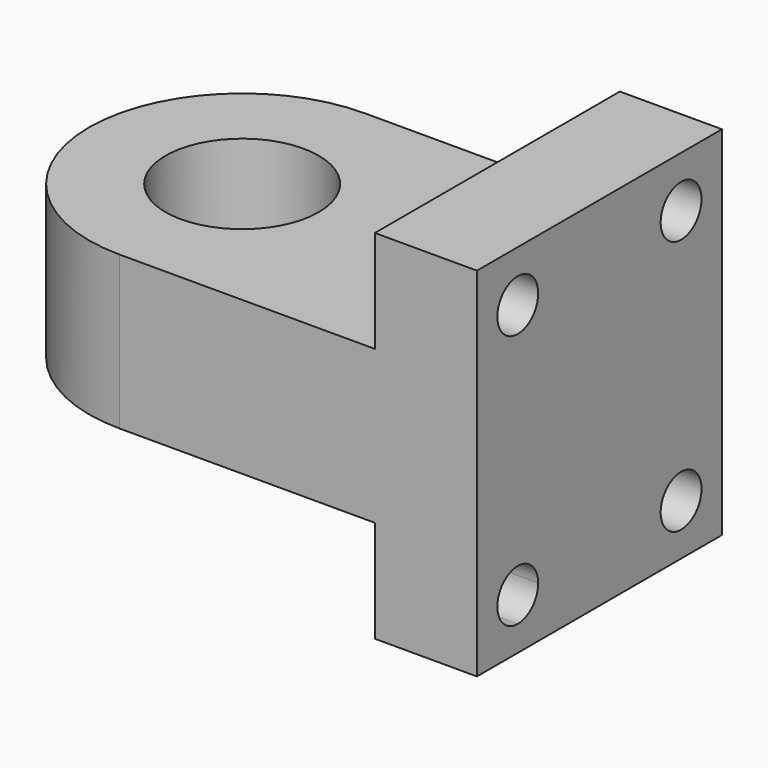
from build123d import *

# Parameters (mm, degrees)
F1_DEPTH = 30
F2_R     = 29.99999
F3_R     = 15
F4_DEPTH = 15
F6_R     = 5
F7_DEPTH = 20


# Not quite as in the source:
# - a fillet or chamfer is up to 0.001 mm smaller than in the source, because OpenCascade refuses the exact size


with BuildPart() as f1:
    # F0 (on Front) → F1 (new body, symmetric)
    with BuildSketch(Plane.XZ):
        Polygon((-100, 0), (0, 0), (0, 35), (-20, 35), (-20, 15), (-100, 15), align=None)
    extrude(amount=F1_DEPTH, both=True)

    # F2 (radius 30 in the source; OpenCascade refuses exactly that, so slightly less here)
    f2_edges = [f1.edges().sort_by_distance(p)[0] for p in [
        (-100, -30, 7.5),
        (-100, 30, 7.5),
    ]]
    fillet(f2_edges, radius=F2_R)

    # F3 (on face) → F4 (cut, through all)
    with BuildSketch(Plane.XY.offset(15)):
        with Locations((-70, 0)):
            Circle(F3_R)
    extrude(amount=-F4_DEPTH, mode=Mode.SUBTRACT)

    # F5: F1 across plane


with BuildPart() as f1_1:
    add(f1.part)
    add(f1.part.mirror(Plane.XY))

    # F6 (on face) → F7 (cut, through all)
    with BuildSketch(Plane.YZ):
        with BuildLine():
            ThreePointArc((-20, -30), (-16.4644660941, -28.5355339059), (-15, -25))
            ThreePointArc((-15, -25), (-23.5355339059, -21.4644660941), (-20, -30))
        make_face()
        with Locations((-20, 25)):
            Circle(F6_R)
        with Locations((20, -25)):
            Circle(F6_R)
        with Locations((20, 25)):
            Circle(F6_R)
    extrude(amount=-F7_DEPTH, mode=Mode.SUBTRACT)


solid = f1_1.part
